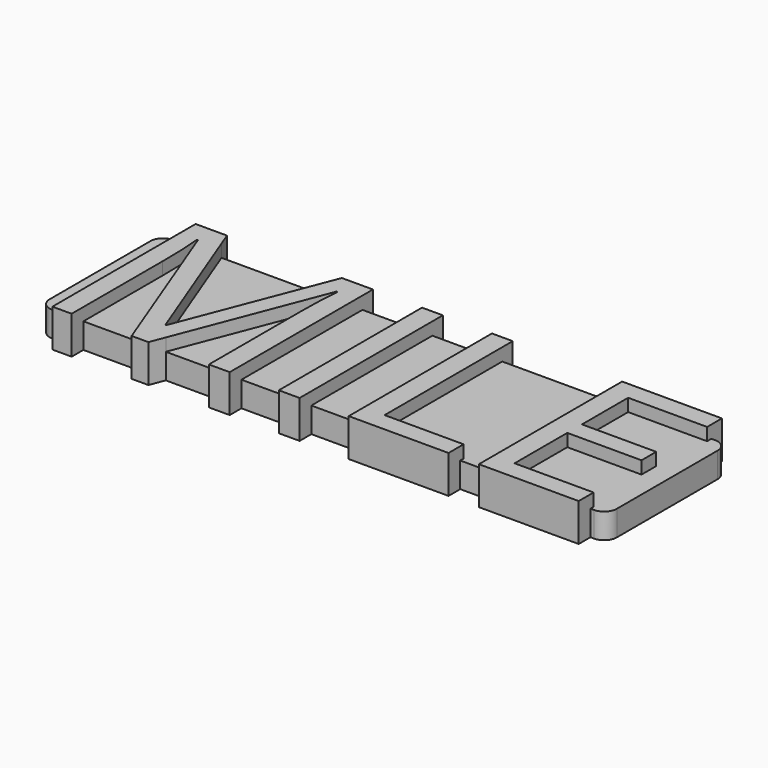
from build123d import *

# Parameters (mm, degrees)
F0_W          = 90
F0_H          = 24
F1_DEPTH      = 4
F2_R          = 2
F3_W          = 3.0530606605
F3_H          = 2.3263783336
F3_W_2        = 3.3017825066
F3_H_2        = 24
F3_H_3        = 2.0838745336
F3_W_3        = 15.8373635484
F4_DEPTH      = 2
F4_DEPTH_BACK = 4
F5_TEXT_SIZE  = 17.3611111111
F6_DEPTH      = 1.5


# Not quite as in the source:
# - Text() gives the source's letters only with a copy of the font that has no kerning and outlines rounded to 1/6400 em; it was checked with that copy


with BuildPart() as f1:
    # F0 (on Top) → F1 (new body)
    with BuildSketch(Plane.XY):
        Rectangle(F0_W, F0_H)
    extrude(amount=F1_DEPTH)

    # F2
    f2_edges = [f1.edges().sort_by_distance(p)[0] for p in [
        (-45, -12, 2),
        (45, 12, 2),
        (-45, 12, 2),
        (45, -12, 2),
    ]]
    fillet(f2_edges, radius=F2_R)

    # F3 (on face) → F4 (join, two sides)
    with BuildSketch(Plane.XY.offset(4)) as f4_sk:
        with Locations((-39.5685366865, -13.1631891668)):
            Rectangle(F3_W, F3_H)
        with BuildLine():
            Line((-38.1601492331, 10.8567085809), (-29.4125200231, -12))
            Line((-29.4125200231, -12), (-24.9617121707, -12))
            Line((-24.9617121707, -12), (-16.1420478099, 10.819400304))
            Line((-16.1420478099, 10.819400304), (-15.9865966561, 10.819400304))
            add(Edge.make_bspline(
                [(-16.2601906867, 3.9795495371), (-16.2601906867, 7.1258808899), (-15.9865966561, 10.819400304)],
                knots=[0, 0, 0, 1, 1, 1], degree=2))
            Line((-16.2601906867, 3.9795495371), (-16.2601906867, -12))
            Line((-16.2601906867, -12), (-12.9584081802, -12))
            Line((-12.9584081802, -12), (-12.9584081802, 12))
            Line((-12.9584081802, 12), (-18.7022157699, 12))
            Line((-18.7022157699, 12), (-26.96766616, -9.3519414122))
            Line((-26.96766616, -9.3519414122), (-27.1231173138, -9.3519414122))
            Line((-27.1231173138, -9.3519414122), (-35.3205859324, 12))
            Line((-35.3205859324, 12), (-41.0950670167, 12))
            Line((-41.0950670167, 12), (-41.0950670167, -12))
            Line((-41.0950670167, -12), (-38.0420063562, -12))
            Line((-38.0420063562, -12), (-38.0420063562, 3.7432637833))
            add(Edge.make_bspline(
                [(-38.3156003869, 10.8567085809), (-38.0420063562, 7.8658283819), (-38.0420063562, 3.7432637833)],
                knots=[0, 0, 0, 1, 1, 1], degree=2))
            Line((-38.3156003869, 10.8567085809), (-38.1601492331, 10.8567085809))
        make_face()
        Polygon((-18.7022157699, 12), (-12.9584081802, 12), (-12.9584081802, 14.0838745336), (-17.8955368247, 14.0838745336), align=None)
        with Locations((-14.6092994335, -13.1631891668)):
            Rectangle(F3_W_2, F3_H)
        with Locations((-3.5163050988, -13.1631891668)):
            Rectangle(F3_W_2, F3_H)
        with Locations((-3.5163050988, 0)):
            Rectangle(F3_W_2, F3_H_2)
        with Locations((-3.5163050988, 13.0419372668)):
            Rectangle(F3_W_2, F3_H_3)
        Polygon((5.9257979826, 12), (5.9257979826, -12), (21.763161531, -12), (21.763161531, -11.3354981346), (9.2275804892, -11.3354981346), (9.2275804892, 12), align=None)
        with Locations((7.5766892359, 13.0419372668)):
            Rectangle(F3_W_2, F3_H_3)
        with Locations((34.5008290728, -13.1631891668)):
            Rectangle(F3_W_3, F3_H)
        Polygon((26.5821472986, 12), (26.5821472986, -12), (42.419510847, -12), (42.419510847, -11.3728064115), (29.8839298052, -11.3728064115), (29.8839298052, -0.9202708305), (41.6609092165, -0.9202708305), (41.6609092165, 1.9959928147), (29.8839298052, 1.9959928147), (29.8839298052, 11.14895675), (42.419510847, 11.14895675), (42.419510847, 12), align=None)
        with Locations((34.5008290728, 13.0419372668)):
            Rectangle(F3_W_3, F3_H_3)
        Polygon((-41.0950670167, 14.0838745336), (-41.0950670167, 12), (-35.3205859324, 12), (-36.1206300953, 14.0838745336), align=None)
        Polygon((-29.4125200231, -12), (-28.5221776979, -14.3263783336), (-25.860853945, -14.3263783336), (-24.9617121707, -12), align=None)
        with Locations((13.8444797568, -13.1631891668)):
            Rectangle(F3_W_3, F3_H)
    extrude(amount=F4_DEPTH)
    extrude(f4_sk.sketch, amount=-F4_DEPTH_BACK)

    # F5 (on face) → F6 (cut)
    with BuildSketch(Plane(origin=(0, 0, 0), x_dir=(1, 0, 0), z_dir=(0, 0, -1))):
        with Locations((-38.2351345486, -6.25)):
            Text('5280 feet', F5_TEXT_SIZE, font='Open Sans', text_align=(TextAlign.LEFT, TextAlign.BOTTOM))
    extrude(amount=-F6_DEPTH, mode=Mode.SUBTRACT)


solid = f1.part
